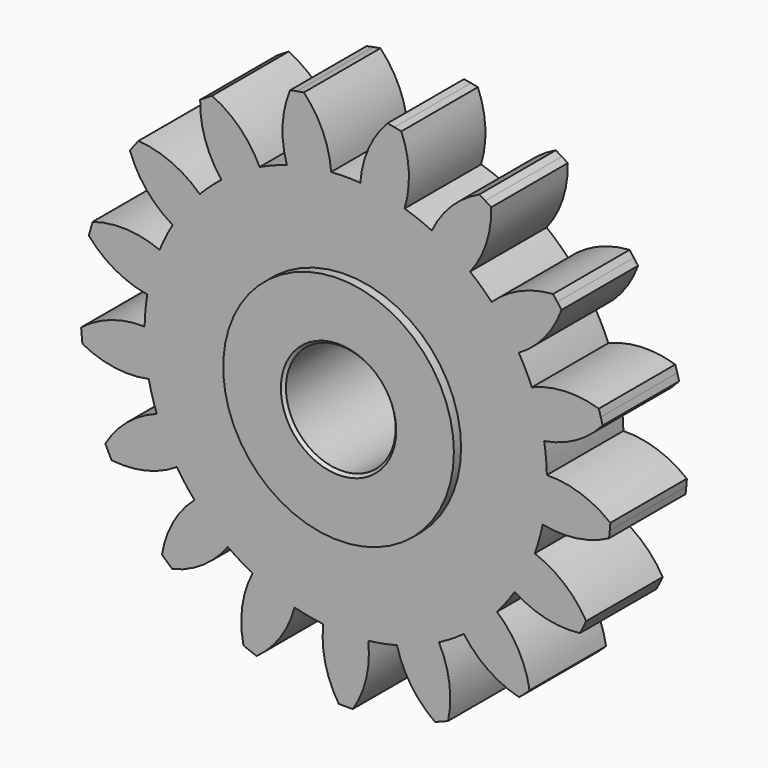
from build123d import *

# Parameters (mm, degrees)
F0_R     = 4.1
F1_DEPTH = 3.4
F0_R_2   = 3.8
F0_R_3   = 1.95
F2_DEPTH = 3.72
F3_DEPTH = 3.28
F4_SIZE  = 0.1
F5_SIZE  = 0.1
F6_SIZE  = 0.1
F7_DEPTH = 3.72


# Not quite as in the source:
# - a feature names something its author has since deleted; it is built from what else it names


with BuildPart() as f1:
    # F0 (on Front) → F1 (new body)
    with BuildSketch(Plane.XZ):
        with BuildLine():
            ThreePointArc((-9.1306946704, 2.3368867827), (-8.1937279785, 1.5734002793), (-7.0529357563, 1.1741367966))
            ThreePointArc((-7.0529357563, 1.1741367966), (-7.1195743604, 0.6589088915), (-7.1486252748, 0.1402022865))
            ThreePointArc((-7.1486252748, 0.1402022865), (-8.3432287104, -0.042236429), (-9.4045806012, -0.6200715414))
            ThreePointArc((-9.4045806012, -0.6200715414), (-9.3954740629, -0.7454476061), (-9.384696163, -0.870691063))
            ThreePointArc((-9.384696163, -0.870691063), (-9.3722488189, -0.9957796327), (-9.3581342447, -1.120691063))
            ThreePointArc((-9.3581342447, -1.120691063), (-8.2085925976, -1.4934044314), (-7.0008156513, -1.4529556828))
            ThreePointArc((-7.0008156513, -1.4529556828), (-6.8768331336, -1.9574641892), (-6.7165444751, -2.4516382918))
            ThreePointArc((-6.7165444751, -2.4516382918), (-7.76441436, -3.053950319), (-8.544935067, -3.9767712658))
            ThreePointArc((-8.544935067, -3.9767712658), (-8.4914364249, -4.0897594601), (-8.43644384, -4.2020281216))
            ThreePointArc((-8.43644384, -4.2020281216), (-8.3799669873, -4.3135574983), (-8.3220158032, -4.4243279682))
            ThreePointArc((-8.3220158032, -4.4243279682), (-7.1152349462, -4.3573127689), (-6.0032028311, -3.8838197394))
            ThreePointArc((-6.0032028311, -3.8838197394), (-5.7053436074, -4.3094726268), (-5.3773631048, -4.7123737159))
            ThreePointArc((-5.3773631048, -4.7123737159), (-6.1368874979, -5.6525550384), (-6.5313316874, -6.7950225452))
            ThreePointArc((-6.5313316874, -6.7950225452), (-6.4406375804, -6.8810473446), (-6.3488105376, -6.9658617383))
            ThreePointArc((-6.3488105376, -6.9658617383), (-6.255866712, -7.0494508071), (-6.1618224526, -7.1317998474))
            ThreePointArc((-6.1618224526, -7.1317998474), (-5.0607335264, -6.6333809478), (-4.1948295471, -5.7901558762))
            ThreePointArc((-4.1948295471, -5.7901558762), (-3.7633208909, -6.0794667424), (-3.3119438366, -6.3366811521))
            ThreePointArc((-3.3119438366, -6.3366811521), (-3.6805479914, -7.487745529), (-3.6356508664, -8.6955544836))
            ThreePointArc((-3.6356508664, -8.6955544836), (-3.5200054468, -8.7430078723), (-3.4037408432, -8.7889233284))
            ThreePointArc((-3.4037408432, -8.7889233284), (-3.2868775071, -8.8332927753), (-3.1694359951, -8.8761084081))
            ThreePointArc((-3.1694359951, -8.8761084081), (-2.3227497605, -8.0135884705), (-1.8199250223, -6.9145045313))
            ThreePointArc((-1.8199250223, -6.9145045313), (-1.3130441845, -7.0284005982), (-0.7992311491, -7.1051903261))
            ThreePointArc((-0.7992311491, -7.1051903261), (-0.727143962, -8.311678782), (-0.2489808346, -9.4217107546))
            ThreePointArc((-0.2489808346, -9.4217107546), (-0.123991383, -9.4241843752), (0.0010198831, -9.4249999448))
            ThreePointArc((0.0010198831, -9.4249999448), (0.1260309698, -9.4241573201), (0.2510198831, -9.4216566494))
            ThreePointArc((0.2510198831, -9.4216566494), (0.7289427654, -8.3115212183), (0.8007688415, -7.1050171895))
            ThreePointArc((0.8007688415, -7.1050171895), (1.3145652461, -7.0281162635), (1.8214214224, -6.9141104997))
            ThreePointArc((1.8214214224, -6.9141104997), (2.3244840135, -8.0130855914), (3.1713568956, -8.8754222683))
            ThreePointArc((3.1713568956, -8.8754222683), (3.2887891386, -8.8325812196), (3.4056428696, -8.7881864821))
            ThreePointArc((3.4056428696, -8.7881864821), (3.5218975334, -8.742245865), (3.6375326803, -8.6947674494))
            ThreePointArc((3.6375326803, -8.6947674494), (3.6821684093, -7.4869488064), (3.3133151488, -6.3359642301))
            ThreePointArc((3.3133151488, -6.3359642301), (3.764636526, -6.078652139), (4.1960825592, -5.7892478921))
            ThreePointArc((4.1960825592, -5.7892478921), (5.0621690097, -6.6322855443), (6.1633657783, -7.1304661337))
            ThreePointArc((6.1633657783, -7.1304661337), (6.2573922134, -7.0480967422), (6.3503179465, -6.9644875604))
            ThreePointArc((6.3503179465, -6.9644875604), (6.4421266315, -6.8796532953), (6.5328021188, -6.7936088699))
            ThreePointArc((6.5328021188, -6.7936088699), (6.1381106848, -5.6512267557), (5.3783828347, -4.7112098322))
            ThreePointArc((5.3783828347, -4.7112098322), (5.7062761334, -4.3082377707), (6.00404323, -3.8825204303))
            ThreePointArc((6.00404323, -3.8825204303), (7.1161845365, -4.3557644871), (8.3229834462, -4.4225073832))
            ThreePointArc((8.3229834462, -4.4225073832), (8.3809053661, -4.3117340184), (8.4373530488, -4.2002022011))
            ThreePointArc((8.4373530488, -4.2002022011), (8.492316565, -4.0879315502), (8.5457862464, -3.9749418147))
            ThreePointArc((8.5457862464, -3.9749418147), (7.7650725635, -3.0522802473), (6.7170749034, -2.4501846343))
            ThreePointArc((6.7170749034, -2.4501846343), (6.8772566086, -1.9559758535), (7.0011299372, -1.4514405265))
            ThreePointArc((7.0011299372, -1.4514405265), (8.2090091905, -1.4913388042), (9.3584507476, -1.1180449923))
            ThreePointArc((9.3584507476, -1.1180449923), (9.3724970598, -0.9934404183), (9.3848843789, -0.868659999))
            ThreePointArc((9.3848843789, -0.868659999), (9.3956105125, -0.7437258211), (9.4046735619, -0.618659999))
            ThreePointArc((9.4046735619, -0.618659999), (8.3432765874, -0.0407321266), (7.1485947646, 0.1417493946))
            ThreePointArc((7.1485947646, 0.1417493946), (7.119431592, 0.6604497002), (7.0526814835, 1.1756631713))
            ThreePointArc((7.0526814835, 1.1756631713), (8.19338727, 1.5751735359), (9.1301887056, 2.3388628005))
            ThreePointArc((9.1301887056, 2.3388628005), (9.0983662855, 2.4597471284), (9.0649434237, 2.5801987762))
            ThreePointArc((9.0649434237, 2.5801987762), (9.0299259996, 2.7001965561), (8.9933201729, 2.8197193598))
            ThreePointArc((8.9933201729, 2.8197193598), (7.794773105, 2.9756140317), (6.6146636541, 2.7145395084))
            ThreePointArc((6.6146636541, 2.7145395084), (6.4000942258, 3.1876784501), (6.1517355927, 3.6439880896))
            ThreePointArc((6.1517355927, 3.6439880896), (7.0710932374, 4.4285897362), (7.6687594725, 5.4791197426))
            ThreePointArc((7.6687594725, 5.4791197426), (7.5954176181, 5.5803455276), (7.5207396972, 5.6805897059))
            ThreePointArc((7.5207396972, 5.6805897059), (7.444738846, 5.7798346442), (7.3674284334, 5.8780628849))
            ThreePointArc((7.3674284334, 5.8780628849), (6.1935005716, 5.5904666436), (5.1873914517, 4.9207184361))
            ThreePointArc((5.1873914517, 4.9207184361), (4.8163943669, 5.2843963991), (4.4199691978, 5.6201754679))
            ThreePointArc((4.4199691978, 5.6201754679), (4.9938151748, 6.683904295), (5.1716286044, 7.8793960795))
            ThreePointArc((5.1716286044, 7.8793960795), (5.0666724743, 7.9472923086), (4.9608250949, 8.0137905749))
            ThreePointArc((4.9608250949, 8.0137905749), (4.8541050851, 8.0788791811), (4.7465312174, 8.1425466779))
            ThreePointArc((4.7465312174, 8.1425466779), (3.7557669795, 7.4503007335), (3.0595379066, 6.4623314522))
            ThreePointArc((3.0595379066, 6.4623314522), (2.5822180472, 6.6674320361), (2.0912654051, 6.8373320093))
            ThreePointArc((2.0912654051, 6.8373320093), (2.2421089696, 8.0365222748), (1.9760667465, 9.2155187165))
            ThreePointArc((1.9760667465, 9.2155187165), (1.8536604305, 9.2409181367), (1.7309279903, 9.2646917538))
            ThreePointArc((1.7309279903, 9.2646917538), (1.6078910188, 9.2868353852), (1.4845711627, 9.307345135))
            ThreePointArc((1.4845711627, 9.307345135), (0.8107889051, 8.3039366723), (0.5184795371, 7.1311765488))
            ThreePointArc((0.5184795371, 7.1311765488), (-0.0006988298, 7.1499999658), (-0.5198735073, 7.1310750618))
            ThreePointArc((-0.5198735073, 7.1310750618), (-0.8124228005, 8.3037784061), (-1.4864122256, 9.307051289))
            ThreePointArc((-1.4864122256, 9.307051289), (-1.609717186, 9.2865190239), (-1.7327389902, 9.2643532204))
            ThreePointArc((-1.7327389902, 9.2643532204), (-1.8554559982, 9.2405577775), (-1.9778466235, 9.2151368809))
            ThreePointArc((-1.9778466235, 9.2151368809), (-2.2436700583, 8.0360880591), (-2.0926019054, 6.8369230846))
            ThreePointArc((-2.0926019054, 6.8369230846), (-2.5835911424, 6.6669000899), (-3.0609364181, 6.4616691531))
            ThreePointArc((-3.0609364181, 6.4616691531), (-3.7573792917, 7.4494877329), (-4.7482933229, 8.141519239))
            ThreePointArc((-4.7482933229, 8.141519239), (-4.8558534091, 8.0778284625), (-4.9625593299, 8.0127167613))
            ThreePointArc((-4.9625593299, 8.0127167613), (-5.0683923152, 7.946195589), (-5.1733337487, 7.8782766469))
            ThreePointArc((-5.1733337487, 7.8782766469), (-4.9952615939, 6.6828233728), (-4.4211854174, 5.6192187629))
            ThreePointArc((-4.4211854174, 5.6192187629), (-4.8175379075, 5.2833539073), (-5.1884562761, 4.9195956613))
            ThreePointArc((-5.1884562761, 4.9195956613), (-6.19471032, 5.5891261102), (-7.3687003961, 5.8764682823))
            ThreePointArc((-7.3687003961, 5.8764682823), (-7.4459895483, 5.7782233123), (-7.521968919, 5.6789619282))
            ThreePointArc((-7.521968919, 5.6789619282), (-7.5966251432, 5.5787015903), (-7.6699450885, 5.477459935))
            ThreePointArc((-7.6699450885, 5.477459935), (-7.0720515108, 4.4270593007), (-6.1525240836, 3.6426566406))
            ThreePointArc((-6.1525240836, 3.6426566406), (-6.4007839559, 3.1862932618), (-6.6152509821, 2.7131078939))
            ThreePointArc((-6.6152509821, 2.7131078939), (-7.7954169073, 2.9739270108), (-8.9939302083, 2.817772952))
            ThreePointArc((-8.9939302083, 2.817772952), (-9.0305101669, 2.6982422288), (-9.0655016202, 2.5782368733))
            ThreePointArc((-9.0655016202, 2.5782368733), (-9.0988984129, 2.4577779948), (-9.1306946704, 2.3368867827))
        make_face()
        Circle(F0_R, mode=Mode.SUBTRACT)
    extrude(amount=F1_DEPTH)



with BuildPart() as f2:
    # F0 (on Front) → F2 (new body)
    with BuildSketch(Plane.XZ):
        Circle(F0_R_2)
        Circle(F0_R_3, mode=Mode.SUBTRACT)
    extrude(amount=F2_DEPTH)

    # F0 (on Front) → F3 (join)
    with BuildSketch(Plane.XZ):
        Circle(F0_R_2)
        Circle(F0_R_3, mode=Mode.SUBTRACT)
    extrude(amount=-F3_DEPTH)

    # F4
    f4_edges = [f2.edges().sort_by_distance(p)[0] for p in [
        (-1.95, 3.28, 0),
    ]]
    chamfer(f4_edges, length=F4_SIZE)

    # F5
    f5_edges = [f2.edges().sort_by_distance(p)[0] for p in [
        (-1.95, -3.72, 0),
    ]]
    chamfer(f5_edges, length=F5_SIZE)

    # F6
    f6_edges = [f2.edges().sort_by_distance(p)[0] for p in [
        (-3.8, 3.28, 0),
    ]]
    chamfer(f6_edges, length=F6_SIZE)


with BuildPart() as f1_1:
    add(f1.part)

    add(f2.part)  # F7 merges F2
    # F0 (on Front) → F7 (join)
    with BuildSketch(Plane.XZ):
        Circle(F0_R)
        Circle(F0_R_2, mode=Mode.SUBTRACT)
    extrude(amount=F7_DEPTH)


solid = f1_1.part
